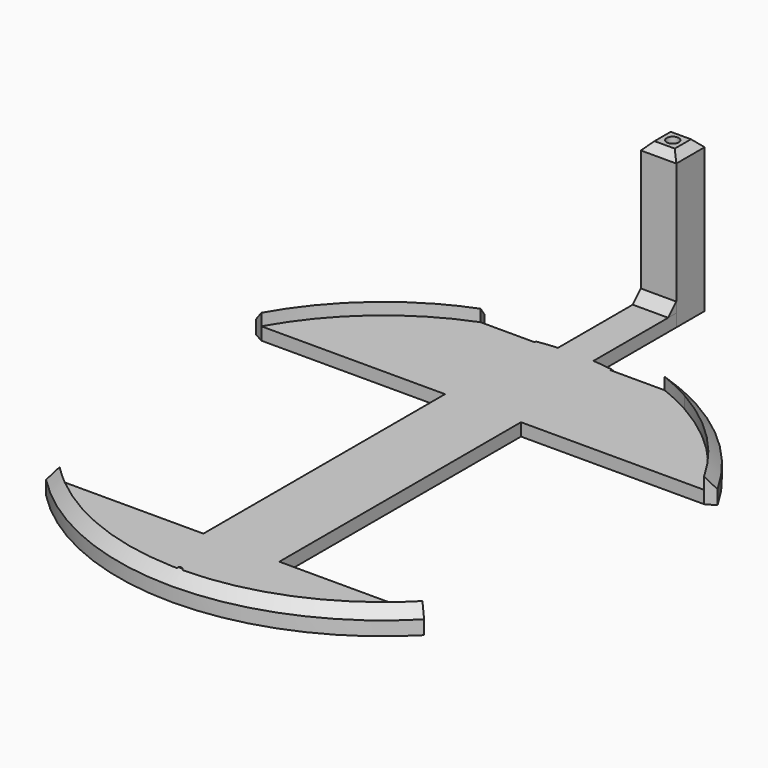
from build123d import *

# Parameters (mm, degrees)
F1_DEPTH     = 5
F2_DEPTH     = 10
F3_DEPTH     = 10
F4_SIZE      = 4.5
F5_T2_ANGLE  = 52.1255505296
F6_DEPTH     = 10
F7_DEPTH     = 10
F8_T2_ANGLE  = 44.4260668477
F9_DEPTH     = 5
F10_DEPTH    = 5
F11_DEPTH    = 5
F12_DEPTH    = 60
F13_T2_ANGLE = 20.3893123961
F14_SIZE     = 4.99999
F15_SIZE     = 4.99999
F16_SIZE     = 3
F18_DEPTH    = 14


# Not quite as in the source:
# - a fillet or chamfer that OpenCascade refuses, or shapes differently, is made with other operations: its cross-section is extruded or revolved along the edge and cut away or added
# - a fillet or chamfer is up to 0.001 mm smaller than in the source, because OpenCascade refuses the exact size


with BuildPart() as f1:
    # F0 (on Top) → F1 (new body)
    with BuildSketch(Plane.XY):
        with BuildLine():
            Line((15.124610185, 49.1284800026), (87.4441676307, 49.1284800026))
            ThreePointArc((87.4441676307, 49.1284800026), (70.8958934178, 70.9497166767), (49.0621045575, 87.481426008))
            ThreePointArc((49.0621045575, 87.481426008), (42.8023254488, 90.7086045322), (36.3315169542, 93.4885601333))
            Line((36.3315169542, 93.4885601333), (15, 93.4885601333))
            Line((15, 93.4885601333), (7, 93.4885601333))
            Line((7, 93.4885601333), (0, 93.4885601333))
            Line((0, 93.4885601333), (-7, 93.4885601333))
            Line((-7, 93.4885601333), (-14.9701492537, 93.4885601333))
            Line((-14.9701492537, 93.4885601333), (-36.3315169542, 93.4885601333))
            ThreePointArc((-36.3315169542, 93.4885601333), (-65.7423699065, 75.7497907527), (-87.4441676307, 49.1284800026))
            Line((-87.4441676307, 49.1284800026), (-14.875389815, 49.1284800026))
            Line((-14.875389815, 49.1284800026), (-14.875389815, -70.1864178667))
            Line((-14.875389815, -70.1864178667), (-71.6516346432, -70.1864178667))
            ThreePointArc((-71.6516346432, -70.1864178667), (-40.4072663325, -91.8005600611), (-3.3654241895, -100.2435230827))
            ThreePointArc((-3.3654241895, -100.2435230827), (-2.227617662, -100.2753201611), (-1.0895229177, -100.2941642982))
            ThreePointArc((-1.0895229177, -100.2941642982), (-1.0617419835, -100.1919997221), (-1.0235513801, -100.0932532857))
            ThreePointArc((-1.0235513801, -100.0932532857), (0.0168897899, -99.4936635029), (0.9104513343, -100.2958938327))
            ThreePointArc((0.9104513343, -100.2958938327), (1.1146686841, -100.2938196477), (1.318881372, -100.2913283985))
            ThreePointArc((1.318881372, -100.2913283985), (39.4683475891, -92.2081316294), (71.6516346432, -70.1864178667))
            Line((71.6516346432, -70.1864178667), (15.124610185, -70.1864178667))
            Line((15.124610185, -70.1864178667), (15.124610185, 49.1284800026))
        make_face()
    extrude(amount=F1_DEPTH)

    # F0 (on Top) → F2 (join)
    with BuildSketch(Plane.XY):
        with BuildLine():
            ThreePointArc((-87.4441676307, 49.1284800026), (-65.7423699065, 75.7497907527), (-36.3315169542, 93.4885601333))
            Line((-36.3315169542, 93.4885601333), (-37.8528765874, 97.4033353333))
            ThreePointArc((-37.8528765874, 97.4033353333), (-68.4952906802, 78.9217660385), (-91.1058376611, 51.1857044893))
            Line((-91.1058376611, 51.1857044893), (-87.4441676307, 49.1284800026))
        make_face()
        with BuildLine():
            Line((74.6520021956, -73.1254303795), (71.6516346432, -70.1864178667))
            ThreePointArc((71.6516346432, -70.1864178667), (39.4683475891, -92.2081316294), (1.318881372, -100.2913283985))
            ThreePointArc((1.318881372, -100.2913283985), (1.1146686841, -100.2938196477), (0.9104513343, -100.2958938327))
            ThreePointArc((0.9104513343, -100.2958938327), (-0.0565525239, -100.3000521496), (-1.0235513801, -100.2948593303))
            ThreePointArc((-1.0235513801, -100.2948593303), (-1.0565372062, -100.2945172548), (-1.0895229177, -100.2941642982))
            ThreePointArc((-1.0895229177, -100.2941642982), (-2.227617662, -100.2753201611), (-3.3654241895, -100.2435230827))
            ThreePointArc((-3.3654241895, -100.2435230827), (-40.4072663325, -91.8005600611), (-71.6516346432, -70.1864178667))
            Line((-71.6516346432, -70.1864178667), (-74.6520021956, -73.1254303795))
            ThreePointArc((-74.6520021956, -73.1254303795), (0, -104.5), (74.6520021956, -73.1254303795))
        make_face()
    extrude(amount=F2_DEPTH)

    # F0 (on Top) → F3 (join)
    with BuildSketch(Plane.XY):
        with BuildLine():
            ThreePointArc((-1.0895229177, -100.2941642982), (-1.0565372062, -100.2945172548), (-1.0235513801, -100.2948593303))
            Line((-1.0235513801, -100.2948593303), (-1.0235513801, -100.0932532857))
            ThreePointArc((-1.0235513801, -100.0932532857), (-1.0617419835, -100.1919997221), (-1.0895229177, -100.2941642982))
        make_face()
        with BuildLine():
            ThreePointArc((-1.0235513801, -100.2948593303), (-0.0565525239, -100.3000521496), (0.9104513343, -100.2958938327))
            ThreePointArc((0.9104513343, -100.2958938327), (0.0168897899, -99.4936635029), (-1.0235513801, -100.0932532857))
            Line((-1.0235513801, -100.0932532857), (-1.0235513801, -100.2948593303))
        make_face()
    extrude(amount=F3_DEPTH)

    # F4
    f4_edges = [f1.edges().sort_by_distance(p)[0] for p in [
        (0, -104.5, 10),
    ]]
    chamfer(f4_edges, length=F4_SIZE)

    # F5: chamfer of 4.5 on 1 edges, made by hand

    # F5_s1 → F5_t2 (revolve, cut)
    with BuildSketch(Plane(origin=(0, 0, 0), x_dir=(0, 0, 1), z_dir=(0.9664139426, 0.2569904503, 0))):
        Polygon((5.5, -104.5), (10, -100), (10, -104.5), align=None)
    revolve(axis=Axis((0, 0, 10), (0, 0, 1)), revolution_arc=F5_T2_ANGLE, mode=Mode.SUBTRACT)

    # F0 (on Top) → F9 (join)
    with BuildSketch(Plane.XY):
        with BuildLine():
            Line((-7, 93.4885601333), (0, 93.4885601333))
            Line((0, 93.4885601333), (0, 100.3))
            ThreePointArc((0, 100.3), (-3.5021354992, 100.238840012), (-7, 100.055434635))
            Line((-7, 100.055434635), (-7, 93.4885601333))
        make_face()
        with BuildLine():
            Line((0, 93.4885601333), (7, 93.4885601333))
            Line((7, 93.4885601333), (7, 97.2463861108))
            Line((7, 97.2463861108), (7, 100.055434635))
            ThreePointArc((7, 100.055434635), (3.5021354992, 100.238840012), (0, 100.3))
            Line((0, 100.3), (0, 93.4885601333))
        make_face()
        with BuildLine():
            ThreePointArc((0, 100.3), (3.5021354992, 100.238840012), (7, 100.055434635))
            Line((7, 100.055434635), (7, 135.9660446667))
            Line((7, 135.9660446667), (0, 135.9660446667))
            Line((0, 135.9660446667), (-7, 135.9660446667))
            Line((-7, 135.9660446667), (-7, 100.055434635))
            ThreePointArc((-7, 100.055434635), (-3.5021354992, 100.238840012), (0, 100.3))
        make_face()
    extrude(amount=F9_DEPTH)

    # F0 (on Top) → F10 (join)
    with BuildSketch(Plane.XY):
        with BuildLine():
            Line((-14.9701492537, 93.4885601333), (-7, 93.4885601333))
            Line((-7, 93.4885601333), (-7, 100.055434635))
            ThreePointArc((-7, 100.055434635), (-10.9938610927, 99.6956619832), (-14.9701492537, 99.1765326643))
            Line((-14.9701492537, 99.1765326643), (-14.9701492537, 93.4885601333))
        make_face()
        with BuildLine():
            Line((7, 93.4885601333), (15, 93.4885601333))
            Line((15, 93.4885601333), (14.9701492537, 99.1765326643))
            ThreePointArc((14.9701492537, 99.1765326643), (10.9938610927, 99.6956619832), (7, 100.055434635))
            Line((7, 100.055434635), (7, 97.2463861108))
            Line((7, 97.2463861108), (7, 93.4885601333))
        make_face()
    extrude(amount=F10_DEPTH)

    # F14 (size 5 in the source; OpenCascade refuses exactly that, so slightly less here)
    f14_edges = [f1.edges().sort_by_distance(p)[0] for p in [
        (-10.993861, 99.695662, 5),
    ]]
    chamfer(f14_edges, length=F14_SIZE)

    # F15 (size 5 in the source; OpenCascade refuses exactly that, so slightly less here)
    f15_edges = [f1.edges().sort_by_distance(p)[0] for p in [
        (10.993861, 99.695662, 5),
    ]]
    chamfer(f15_edges, length=F15_SIZE)


with BuildPart() as f6:
    # F0 (on Top) → F6 (new body)
    with BuildSketch(Plane.XY):
        with BuildLine():
            ThreePointArc((36.3315169542, 93.4885601333), (42.8023254488, 90.7086045322), (49.0621045575, 87.481426008))
            Line((49.0621045575, 87.481426008), (50.5608916452, 91.454066263))
            ThreePointArc((50.5608916452, 91.454066263), (44.3068510943, 94.6422365866), (37.8528765874, 97.4033353333))
            Line((37.8528765874, 97.4033353333), (37.0921967708, 95.4459477333))
            Line((37.0921967708, 95.4459477333), (36.3315169542, 93.4885601333))
        make_face()
    extrude(amount=F6_DEPTH)

    # F13: chamfer of 4.5 on 1 edges, made by hand

    # F13_s1 → F13_t2 (revolve, cut)
    with BuildSketch(Plane(origin=(0, 0, 0), x_dir=(0, 0, 1), z_dir=(0.8163257049, -0.5775918485, 0))):
        Polygon((10, -100), (5.5, -104.5), (10, -104.5), align=None)
    revolve(axis=Axis((0, 0, 10), (0, 0, 1)), revolution_arc=F13_T2_ANGLE, mode=Mode.SUBTRACT)


with BuildPart() as f7:
    # F0 (on Top) → F7 (new body)
    with BuildSketch(Plane.XY):
        with BuildLine():
            ThreePointArc((49.0621045575, 87.481426008), (70.8958934178, 70.9497166767), (87.4441676307, 49.1284800026))
            Line((87.4441676307, 49.1284800026), (91.1058376611, 51.1857044893))
            ThreePointArc((91.1058376611, 51.1857044893), (73.6393290849, 74.1451226442), (50.5608916452, 91.454066263))
            Line((50.5608916452, 91.454066263), (49.0621045575, 87.481426008))
        make_face()
    extrude(amount=F7_DEPTH)

    # F8: chamfer of 4.5 on 1 edges, made by hand

    # F8_s1 → F8_t2 (revolve, cut)
    with BuildSketch(Plane(origin=(0, 0, 0), x_dir=(0, 0, 1), z_dir=(0.3904589739, -0.9206203287, 0))):
        Polygon((5.5, -104.5), (10, -100), (10, -104.5), align=None)
    revolve(axis=Axis((0, 0, 10), (0, 0, 1)), revolution_arc=F8_T2_ANGLE, mode=Mode.SUBTRACT)


with BuildPart() as f11:
    # F0 (on Top) → F11 (new body)
    with BuildSketch(Plane.XY):
        with BuildLine():
            ThreePointArc((2.38125, 142.9660446667), (-1.6837980227, 144.6498426894), (0, 140.5847946667))
            ThreePointArc((0, 140.5847946667), (1.6837980227, 141.282246644), (2.38125, 142.9660446667))
        make_face()
    extrude(amount=F11_DEPTH)


with BuildPart() as f12:
    # F0 (on Top) → F12 (new body)
    with BuildSketch(Plane.XY):
        Polygon((0, 135.9660446667), (7, 135.9660446667), (7, 149.9660446667), (-7, 149.9660446667), (-7, 135.9660446667), align=None)
        with BuildLine():
            ThreePointArc((2.38125, 142.9660446667), (1.6837980227, 141.282246644), (0, 140.5847946667))
            ThreePointArc((0, 140.5847946667), (-1.6837980227, 144.6498426894), (2.38125, 142.9660446667))
        make_face(mode=Mode.SUBTRACT)
    extrude(amount=F12_DEPTH)

    # F16
    f16_edges = [f12.edges().sort_by_distance(p)[0] for p in [
        (0, 135.966045, 60),
        (7, 142.966045, 60),
        (0, 149.966045, 60),
        (-7, 142.966045, 60),
    ]]
    chamfer(f16_edges, length=F16_SIZE)


with BuildPart() as f18:
    # F17 (on face) → F18 (new body)
    with BuildSketch(Plane.YZ.offset(7)):
        Polygon((131.9660446667, 5), (135.9660446667, 5), (135.9660446667, 9), align=None)
    extrude(amount=-F18_DEPTH)


solid = Compound([f1.part, f6.part, f7.part, f11.part, f12.part, f18.part])
